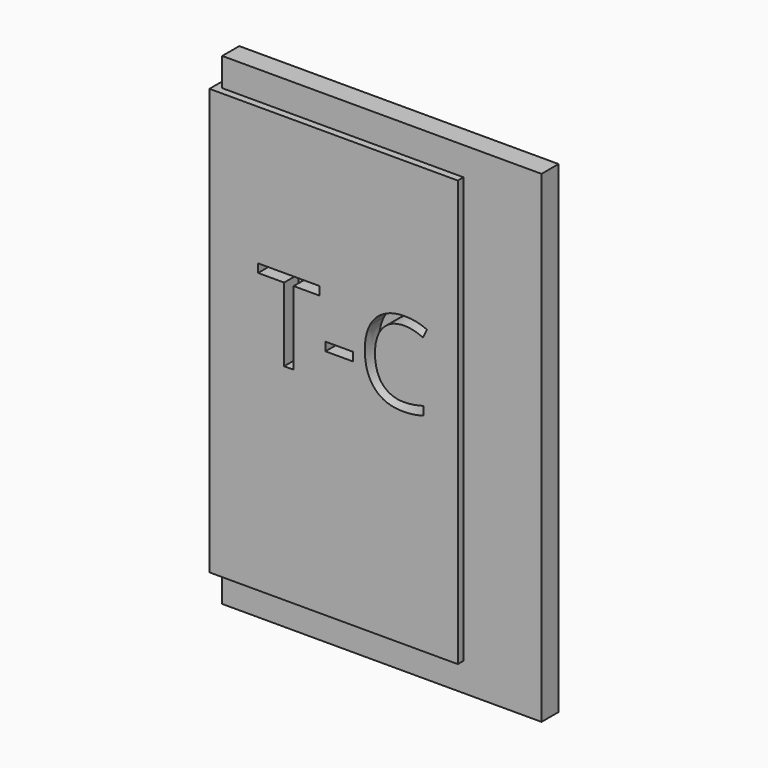
from build123d import *

# Parameters (mm, degrees)
F1_DEPTH     = 1.5
F0_W         = 3.8867378872
F0_H         = 1.2035205322
F2_DEPTH     = 2.5
F0_TEXT_SIZE = 16.215855592
F3_DEPTH     = 2.5


# Not quite as in the source:
# - Text() gives the source's letters only with a copy of the font that has no kerning and outlines rounded to 1/6400 em; it was checked with that copy


with BuildPart() as f1:
    # F0 (on Front) → F1 (new body, symmetric)
    with BuildSketch(Plane.XZ):
        Polygon((80.9848383069, 19.7757222056), (35.9848383069, 19.7757222056), (35.9848383069, 15.7757222056), (69.9848383069, 15.7757222056), (69.9848383069, -44.2242777944), (35.9848383069, -44.2242777944), (35.9848383069, -48.2242777944), (80.9848383069, -48.2242777944), align=None)
    extrude(amount=F1_DEPTH, both=True)

    # F0 (on Front) → F2 (join, symmetric)
    with BuildSketch(Plane.XZ):
        Polygon((69.9848383069, 15.7757222056), (35.9848383069, 15.7757222056), (34.9848383069, 15.7757222056), (34.9848383069, -44.2242777944), (35.9848383069, -44.2242777944), (69.9848383069, -44.2242777944), align=None)
        Polygon((46.8511447198, -4.8428162185), (46.8511447198, -15.2234975249), (45.5057354511, -15.2234975249), (45.5057354511, -4.8428162185), (41.8394318509, -4.8428162185), (41.8394318509, -3.6468968686), (50.51744832, -3.6468968686), (50.51744832, -4.8428162185), align=None, mode=Mode.SUBTRACT)
        with Locations((53.2792112255, -10.876888108)):
            Rectangle(F0_W, F0_H, mode=Mode.SUBTRACT)
        with BuildLine():
            add(Edge.make_bspline(
                [(65.0635775316, -5.3014208845), (63.7485729922, -4.6857251175), (62.4335684527, -4.6857251175)],
                knots=[0, 0, 0, 1, 1, 1], degree=2))
            add(Edge.make_bspline(
                [(62.4335684527, -4.6857251175), (60.5256716932, -4.6857251175), (59.420966531, -5.9563894268)],
                knots=[0, 0, 0, 1, 1, 1], degree=2))
            add(Edge.make_bspline(
                [(59.420966531, -5.9563894268), (58.3162613688, -7.227053736), (58.3162613688, -9.4364640605)],
                knots=[0, 0, 0, 1, 1, 1], degree=2))
            add(Edge.make_bspline(
                [(58.3162613688, -9.4364640605), (58.3162613688, -11.7066838433), (59.3816937558, -12.9469434234)],
                knots=[0, 0, 0, 1, 1, 1], degree=2))
            add(Edge.make_bspline(
                [(59.3816937558, -12.9469434234), (60.4471261427, -14.1872030034), (62.4183660881, -14.1872030034)],
                knots=[0, 0, 0, 1, 1, 1], degree=2))
            add(Edge.make_bspline(
                [(62.4183660881, -14.1872030034), (63.6294878026, -14.1872030034), (65.1826627211, -13.7514018844)],
                knots=[0, 0, 0, 1, 1, 1], degree=2))
            Line((65.1826627211, -13.7514018844), (65.1826627211, -14.9295851423))
            add(Edge.make_bspline(
                [(65.1826627211, -14.9295851423), (63.9791421889, -15.3831223533), (62.2131341658, -15.3831223533)],
                knots=[0, 0, 0, 1, 1, 1], degree=2))
            add(Edge.make_bspline(
                [(62.2131341658, -15.3831223533), (59.6566031826, -15.3831223533), (58.2668536838, -13.8299474349)],
                knots=[0, 0, 0, 1, 1, 1], degree=2))
            add(Edge.make_bspline(
                [(58.2668536838, -13.8299474349), (56.877104185, -12.2767725165), (56.877104185, -9.4187279684)],
                knots=[0, 0, 0, 1, 1, 1], degree=2))
            add(Edge.make_bspline(
                [(56.877104185, -9.4187279684), (56.877104185, -7.6299163984), (57.5460082282, -6.2845071297)],
                knots=[0, 0, 0, 1, 1, 1], degree=2))
            add(Edge.make_bspline(
                [(57.5460082282, -6.2845071297), (58.2149122714, -4.9390978611), (59.4779753983, -4.2106512232)],
                knots=[0, 0, 0, 1, 1, 1], degree=2))
            add(Edge.make_bspline(
                [(59.4779753983, -4.2106512232), (60.7410385253, -3.4822045853), (62.4513045448, -3.4822045853)],
                knots=[0, 0, 0, 1, 1, 1], degree=2))
            add(Edge.make_bspline(
                [(62.4513045448, -3.4822045853), (64.270520844, -3.4822045853), (65.6336662047, -4.1460411735)],
                knots=[0, 0, 0, 1, 1, 1], degree=2))
            Line((65.6336662047, -4.1460411735), (65.0635775316, -5.3014208845))
        make_face(mode=Mode.SUBTRACT)
    extrude(amount=F2_DEPTH, both=True)

    # F0 (on Front) → F3 (join)
    with BuildSketch(Plane.XZ):
        with Locations((41.6975431144, -15.2234975249)):
            Text('T-C', F0_TEXT_SIZE, font='Open Sans', text_align=(TextAlign.LEFT, TextAlign.BOTTOM))
    extrude(amount=-F3_DEPTH)


solid = f1.part
